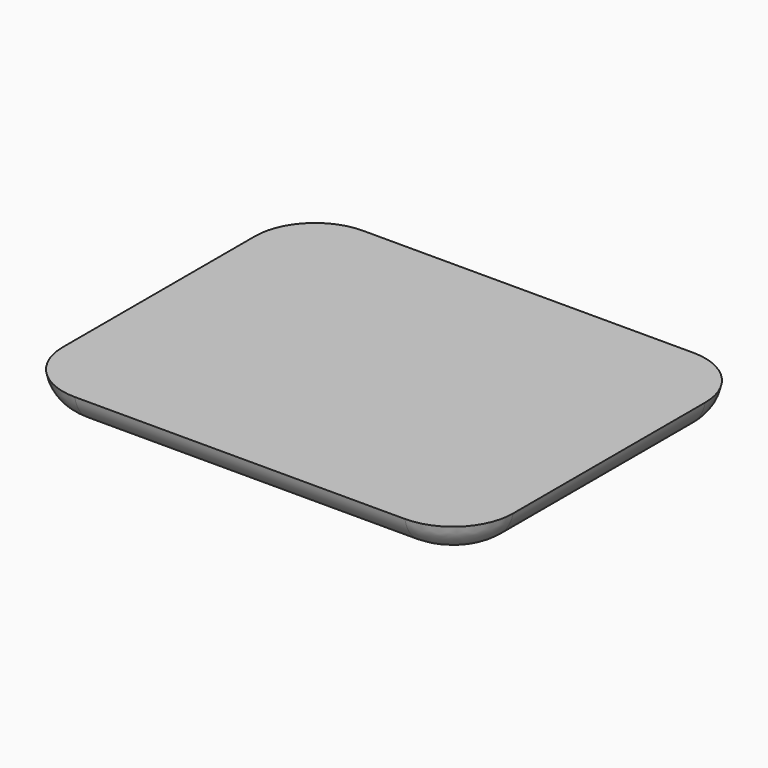
from build123d import *

# Parameters (mm, degrees)
F1_DEPTH     = 25.4
F2_T1_DEPTH  = 279.4
F2_T3_DEPTH  = 203.2
F2_T6_ANGLE  = 90
F2_T8_ANGLE  = 90
F2_T10_ANGLE = 90
F2_T12_ANGLE = 90


# Not quite as in the source:
# - a fillet or chamfer that OpenCascade refuses, or shapes differently, is made with other operations: its cross-section is extruded or revolved along the edge and cut away or added


with BuildPart() as f1:
    # F0 (on Top) → F1 (new body)
    with BuildSketch(Plane.XY):
        with BuildLine():
            Line((-139.7, -152.4), (139.7, -152.4))
            ThreePointArc((139.7, -152.4), (175.6210244843, -137.5210244843), (190.5, -101.6))
            Line((190.5, -101.6), (190.5, 101.6))
            ThreePointArc((190.5, 101.6), (175.6210244843, 137.5210244843), (139.7, 152.4))
            Line((139.7, 152.4), (-139.7, 152.4))
            ThreePointArc((-139.7, 152.4), (-175.6210244843, 137.5210244843), (-190.5, 101.6))
            Line((-190.5, 101.6), (-190.5, -101.6))
            ThreePointArc((-190.5, -101.6), (-175.6210244843, -137.5210244843), (-139.7, -152.4))
        make_face()
    extrude(amount=F1_DEPTH)

    # F2: fillet of radius 30.48 on 1 edges, made by hand

    # F2_s2 → F2_t1 (cut)
    with BuildSketch(Plane.YZ.offset(-139.7)):
        with BuildLine():
            ThreePointArc((-152.4, 25.4), (-142.0210701006, 7.2005154696), (-122.3463147019, 0))
            Line((-122.3463147019, 0), (-152.4, 0))
            Line((-152.4, 0), (-152.4, 25.4))
        make_face()
        with BuildLine():
            ThreePointArc((152.4, 25.4), (142.0210701006, 7.2005154696), (122.3463147019, 0))
            Line((122.3463147019, 0), (152.4, 0))
            Line((152.4, 0), (152.4, 25.4))
        make_face()
    extrude(amount=F2_T1_DEPTH, mode=Mode.SUBTRACT)

    # F2_s4 → F2_t3 (cut)
    with BuildSketch(Plane.XZ.offset(-101.6)):
        with BuildLine():
            ThreePointArc((190.5, 25.4), (180.1210701006, 7.2005154696), (160.4463147019, 0))
            Line((160.4463147019, 0), (190.5, 0))
            Line((190.5, 0), (190.5, 25.4))
        make_face()
        with BuildLine():
            ThreePointArc((-190.5, 25.4), (-180.1210701006, 7.2005154696), (-160.4463147019, 0))
            Line((-160.4463147019, 0), (-190.5, 0))
            Line((-190.5, 0), (-190.5, 25.4))
        make_face()
    extrude(amount=F2_T3_DEPTH, mode=Mode.SUBTRACT)

    # F2_s5 → F2_t6 (revolve, cut)
    with BuildSketch(Plane.XZ.offset(101.6)):
        with BuildLine():
            ThreePointArc((-190.5, 25.4), (-180.1210701006, 7.2005154696), (-160.4463147019, 0))
            Line((-160.4463147019, 0), (-190.5, 0))
            Line((-190.5, 0), (-190.5, 25.4))
        make_face()
    revolve(axis=Axis((-139.7, -101.6, 0), (0, 0, 1)), revolution_arc=F2_T6_ANGLE, mode=Mode.SUBTRACT)

    # F2_s7 → F2_t8 (revolve, cut)
    with BuildSketch(Plane.YZ.offset(139.7)):
        with BuildLine():
            ThreePointArc((-152.4, 25.4), (-142.0210701006, 7.2005154696), (-122.3463147019, 0))
            Line((-122.3463147019, 0), (-152.4, 0))
            Line((-152.4, 0), (-152.4, 25.4))
        make_face()
    revolve(axis=Axis((139.7, -101.6, 0), (0, 0, 1)), revolution_arc=F2_T8_ANGLE, mode=Mode.SUBTRACT)

    # F2_s9 → F2_t10 (revolve, cut)
    with BuildSketch(Plane.XZ.offset(-101.6)):
        with BuildLine():
            ThreePointArc((190.5, 25.4), (180.1210701006, 7.2005154696), (160.4463147019, 0))
            Line((160.4463147019, 0), (190.5, 0))
            Line((190.5, 0), (190.5, 25.4))
        make_face()
    revolve(axis=Axis((139.7, 101.6, 0), (0, 0, 1)), revolution_arc=F2_T10_ANGLE, mode=Mode.SUBTRACT)

    # F2_s11 → F2_t12 (revolve, cut)
    with BuildSketch(Plane.YZ.offset(-139.7)):
        with BuildLine():
            ThreePointArc((152.4, 25.4), (142.0210701006, 7.2005154696), (122.3463147019, 0))
            Line((122.3463147019, 0), (152.4, 0))
            Line((152.4, 0), (152.4, 25.4))
        make_face()
    revolve(axis=Axis((-139.7, 101.6, 0), (0, 0, 1)), revolution_arc=F2_T12_ANGLE, mode=Mode.SUBTRACT)


solid = f1.part
